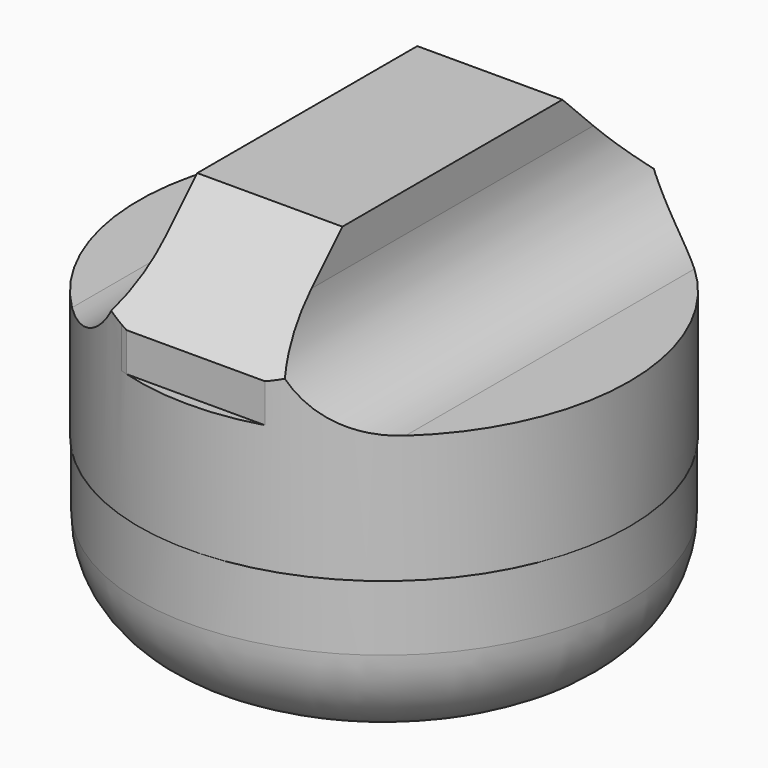
from build123d import *

# Parameters (mm, degrees)
F0_R         = 12.625
F0_R_2       = 10.375
F0_R_3       = 5
F1_DEPTH     = 15
F2_DEPTH     = 15
F3_R         = 12.6739646699
F4_DEPTH     = 6.6
F6_DEPTH     = 7
F7_T4_DEPTH  = 36.6039255786
F7_S5_R      = 12.6739646699
F7_T6_DEPTH  = 20
F7_T10_DEPTH = 24.210816556
F7_S11_R     = 12.6739646699
F7_T12_DEPTH = 14
F8_T1_DEPTH  = 32.8699146781
F9_T1_DEPTH  = 33.2150521969
F10_R        = 5


# Not quite as in the source:
# - a fillet or chamfer that OpenCascade refuses, or shapes differently, is made with other operations: its cross-section is extruded or revolved along the edge and cut away or added
# - a feature names something its author has since deleted; it is built from what else it names


with BuildPart() as f1:
    # F0 (on Top) → F1 (new body)
    with BuildSketch(Plane.XY):
        Circle(F0_R)
        Circle(F0_R_2, mode=Mode.SUBTRACT)
        Circle(F0_R_2)
        Circle(F0_R_3, mode=Mode.SUBTRACT)
    extrude(amount=F1_DEPTH)

    # F0 (on Top) → F2 (join)
    with BuildSketch(Plane.XY):
        Circle(F0_R_3)
        with BuildLine():
            ThreePointArc((2.304625, 2.1105280404), (2.9126944678, 1.1321819366), (3.125, 0))
            ThreePointArc((3.125, 0), (-1.1321819366, -2.9126944678), (-2.304625, 2.1105280404))
            ThreePointArc((-2.304625, 2.1105280404), (0, 3.125), (2.304625, 2.1105280404))
        make_face(mode=Mode.SUBTRACT)
        with BuildLine():
            Line((-2.304625, 2.1105280404), (2.304625, 2.1105280404))
            ThreePointArc((2.304625, 2.1105280404), (0, 3.125), (-2.304625, 2.1105280404))
        make_face()
    extrude(amount=F2_DEPTH)

    # F3 (on face) → F4 (join)
    with BuildSketch(Plane.XY.offset(15)):
        Circle(F3_R)
    extrude(amount=-F4_DEPTH)

    # F5 (on face) → F6 (join)
    with BuildSketch(Plane.XY.offset(15)):
        with BuildLine():
            Line((3.5765423992, 12.0519627893), (-3.921679918, 12.0519627893))
            Line((-3.921679918, 12.0519627893), (-3.921679918, -12.0519627893))
            ThreePointArc((-3.921679918, -12.0519627893), (-3.7494920856, -12.1066382433), (-3.5765423992, -12.1588537667))
            Line((-3.5765423992, -12.1588537667), (3.5765423992, -12.1588537667))
            Line((3.5765423992, -12.1588537667), (3.5765423992, 12.0519627893))
        make_face()
    extrude(amount=F6_DEPTH)

    # F7: fillet of radius 5 on 2 edges, made by hand


with BuildPart() as f7_tool2:
    # F7_s3 → F7_t4 (new body)
    with BuildSketch(Plane.XZ.offset(-12.0519627893)):
        with BuildLine():
            ThreePointArc((-8.921679918, 15), (-5.3861460121, 16.4644660941), (-3.921679918, 20))
            Line((-3.921679918, 20), (-3.921679918, 15))
            Line((-3.921679918, 15), (-8.921679918, 15))
        make_face()
    extrude(amount=F7_T4_DEPTH)

    # F7_s5 → F7_t6 (intersect, symmetric)
    with BuildSketch(Plane.XY.offset(17.5)):
        Circle(F7_S5_R)
    extrude(amount=F7_T6_DEPTH, both=True, mode=Mode.INTERSECT)


with BuildPart() as f1_1:
    add(f1.part)

    # F7_t1: union F7_tool2
    add(f7_tool2.part)


with BuildPart() as f7_tool8:
    # F7_s9 → F7_t10 (new body)
    with BuildSketch(Plane.XZ.offset(12.1588537667)):
        with BuildLine():
            ThreePointArc((8.5765423992, 15), (5.0410084933, 16.4644660941), (3.5765423992, 20))
            Line((3.5765423992, 20), (3.5765423992, 15))
            Line((3.5765423992, 15), (8.5765423992, 15))
        make_face()
    extrude(amount=-F7_T10_DEPTH)

    # F7_s11 → F7_t12 (intersect, symmetric)
    with BuildSketch(Plane.XY.offset(17.5)):
        Circle(F7_S11_R)
    extrude(amount=F7_T12_DEPTH, both=True, mode=Mode.INTERSECT)


with BuildPart() as f1_2:
    add(f1_1.part)

    # F7_t7: union F7_tool8
    add(f7_tool8.part)

    # F8: chamfer of 5 on 1 edges, made by hand

    # F8_s2 → F8_t1 (cut)
    with BuildSketch(Plane.YZ.offset(-16.434957339)):
        Polygon((-12.1588537667, 17), (-7.1588537667, 22), (-12.1588537667, 22), align=None)
    extrude(amount=F8_T1_DEPTH, mode=Mode.SUBTRACT)

    # F9: chamfer of 5 on 1 edges, made by hand

    # F9_s2 → F9_t1 (cut)
    with BuildSketch(Plane.YZ.offset(-16.7800948578)):
        Polygon((12.0519627893, 17), (7.0519627893, 22), (12.0519627893, 22), align=None)
    extrude(amount=F9_T1_DEPTH, mode=Mode.SUBTRACT)

    # F10
    f10_edges = [f1_2.edges().sort_by_distance(p)[0] for p in [
        (-12.625, 0, 0),
    ]]
    fillet(f10_edges, radius=F10_R)


solid = f1_2.part
